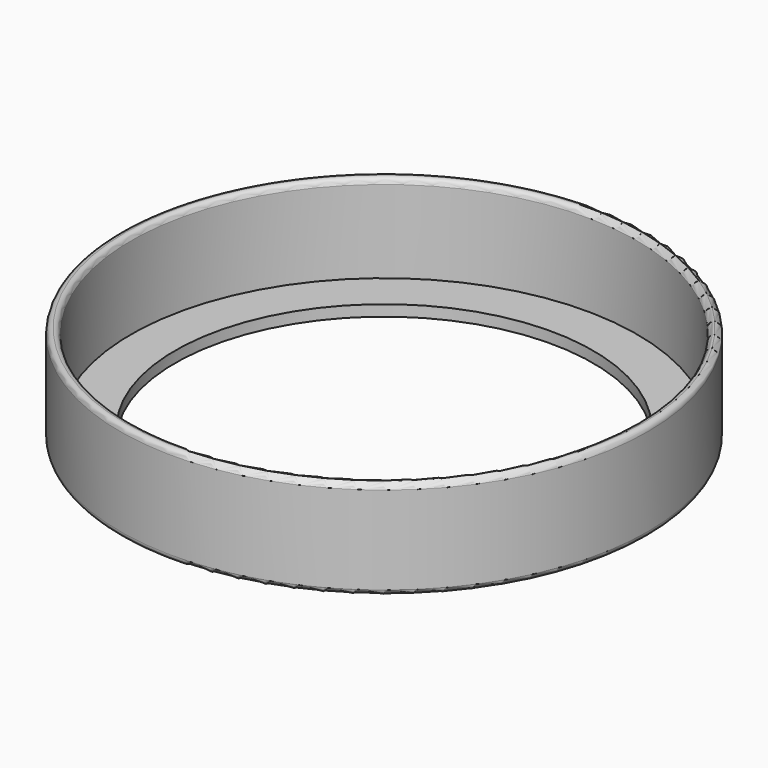
from build123d import *

# Parameters (mm, degrees)
F0_R     = 24
F0_R_2   = 23
F1_DEPTH = 9
F0_R_3   = 19
F2_DEPTH = 1
F3_R     = 0.49999


# Not quite as in the source:
# - a fillet or chamfer is up to 0.001 mm smaller than in the source, because OpenCascade refuses the exact size


with BuildPart() as f1:
    # F0 (on Top) → F1 (new body)
    with BuildSketch(Plane.XY):
        Circle(F0_R)
        Circle(F0_R_2, mode=Mode.SUBTRACT)
    extrude(amount=F1_DEPTH)

    # F0 (on Top) → F2 (join)
    with BuildSketch(Plane.XY):
        Circle(F0_R_2)
        Circle(F0_R_3, mode=Mode.SUBTRACT)
    extrude(amount=F2_DEPTH)

    # F3 (radius 0.5 in the source; OpenCascade refuses exactly that, so slightly less here)
    f3_edges = [f1.edges().sort_by_distance(p)[0] for p in [
        (-24, 0, 0),
        (-24, 0, 9),
        (-23, 0, 9),
    ]]
    fillet(f3_edges, radius=F3_R)


solid = f1.part
